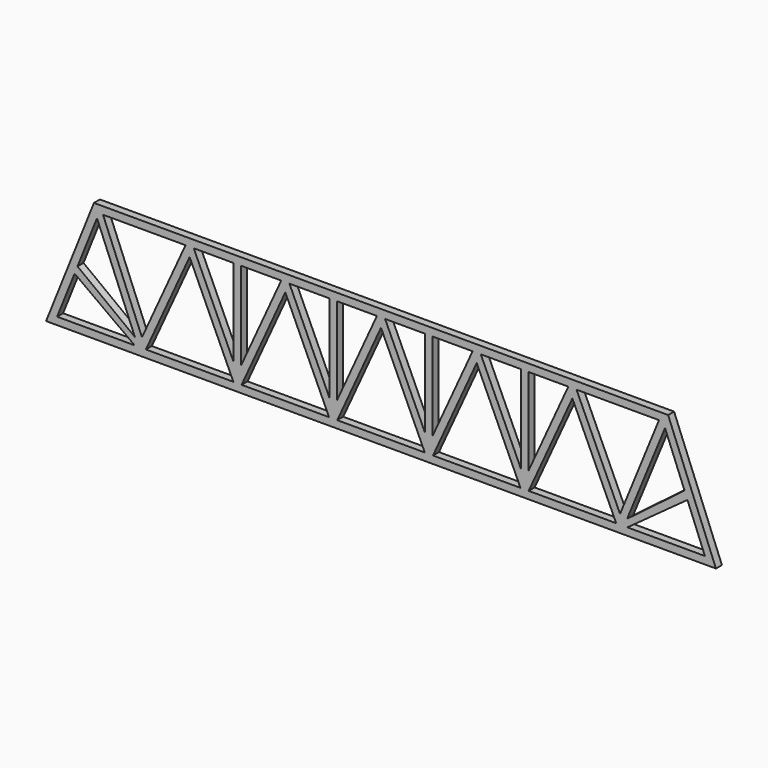
from build123d import *

# Parameters (mm, degrees)
F1_DEPTH = 3.175
F3_W     = 3.175
F3_H     = 50.8
F4_DEPTH = 3.175
F6_DEPTH = 3.175


# Not quite as in the source:
# - a length typed as a fraction of an inch, garbled in the dataset ("3 / 203.2 mm" for 3/8 in), is restored


with BuildPart() as f1:
    # F0 (on Front) → F1 (new body)
    with BuildSketch(Plane.XZ):
        Polygon((-100.2748559753, 0), (0, 0), (0, 3.175), (-18.5744864726, 3.175), (0, 43.8066891587), (0, 47.625), (0, 50.8), (-121.92, 50.8), (-132.0796890642, 25.4007773395), (-140.97, 3.175), (-142.24, 0), align=None)
        Polygon((-104.6410501003, 3.175), (-137.5504203475, 3.175), (-130.1349730994, 21.7136181201), align=None, mode=Mode.SUBTRACT)
        Polygon((-62.7055135274, 3.175), (-99.8544864726, 3.175), (-81.28, 43.8066891587), align=None, mode=Mode.SUBTRACT)
        Polygon((-40.64, 43.8066891587), (-22.0655135274, 3.175), (-59.2144864726, 3.175), align=None, mode=Mode.SUBTRACT)
        Polygon((-128.8950878765, 24.8133311775), (-120.6186164373, 45.5045097755), (-104.527521639, 6.3479696325), align=None, mode=Mode.SUBTRACT)
        Polygon((-101.5186177981, 7.1713344078), (-118.0554031391, 47.625), (-83.0255135274, 47.625), align=None, mode=Mode.SUBTRACT)
        Polygon((-60.96, 6.9933108413), (-79.5344864726, 47.625), (-42.3855135274, 47.625), align=None, mode=Mode.SUBTRACT)
        Polygon((-38.8944864726, 47.625), (-1.7455135274, 47.625), (-20.32, 6.9933108413), align=None, mode=Mode.SUBTRACT)
    extrude(amount=F1_DEPTH)

    # F2: F1 across face


with BuildPart() as f1_1:
    add(f1.part)
    add(f1.part.mirror(Plane(origin=(0, -1.5875, 47.3033445794), x_dir=(0, 1, 0), z_dir=(1, 0, 0))))

    # F3 (on Front) → F4 (join)
    with BuildSketch(Plane.XZ):
        with Locations((-60.96, 25.4)):
            Rectangle(F3_W, F3_H)
        with Locations((-20.32, 25.4)):
            Rectangle(F3_W, F3_H)
        with Locations((60.96, 25.4)):
            Rectangle(F3_W, F3_H)
        Polygon((22.0655135274, 0), (21.9075, 6.9933108413), (21.9075, 50.8), (18.7325, 50.8), (18.7325, 0), align=None)
    extrude(amount=F4_DEPTH)


with BuildPart() as f6:
    # F5 (on Front) → F6 (new body)
    with BuildSketch(Plane.XZ):
        Polygon((14.0807485003, -20.7951998672), (-43.0692514997, -20.7951998672), (-43.0692514997, -23.9701998672), (-39.8942514997, -23.9701998672), (-39.8942514997, -27.1451998672), (10.9057485003, -27.1451998672), (10.9057485003, -23.9701998672), (14.0807485003, -23.9701998672), align=None)
    extrude(amount=F6_DEPTH)


solid = f1_1.part
